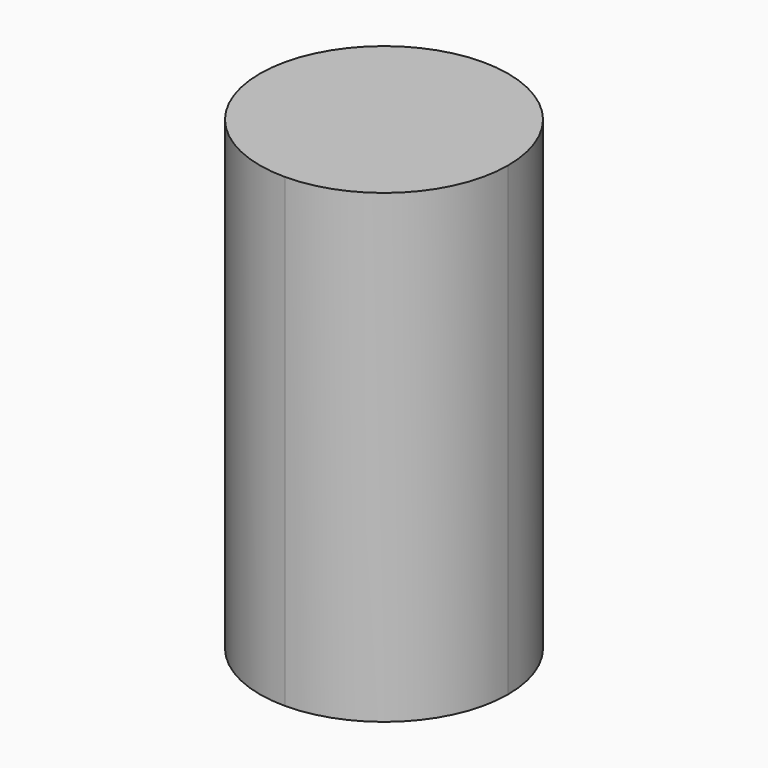
from build123d import *

# Parameters (mm, degrees)
F1_DEPTH = 3


# Not quite as in the source:
# - the program builds the solid bodies; features that only make, move or delete a surface that nothing else refers to are left out


with BuildPart() as f1:
    # F0 (on Top) → F1 (new body)
    with BuildSketch(Plane.XY):
        with BuildLine():
            ThreePointArc((-31.8330490828, 14.4346580839), (-32.631624583, 13.6332361161), (-31.8302026152, 12.8346606159))
            Line((-31.8302026152, 12.8346606159), (-31.8330490828, 14.4346580839))
        make_face()
        with BuildLine():
            Line((-31.8330490828, 14.4346580839), (-31.8302026152, 12.8346606159))
            ThreePointArc((-31.8302026152, 12.8346606159), (-31.2654374585, 13.0694773381), (-31.031625849, 13.6346593499))
            ThreePointArc((-31.031625849, 13.6346593499), (-31.2664438372, 14.2008477404), (-31.8330490828, 14.4346580839))
        make_face()
    extrude(amount=F1_DEPTH)


solid = f1.part
